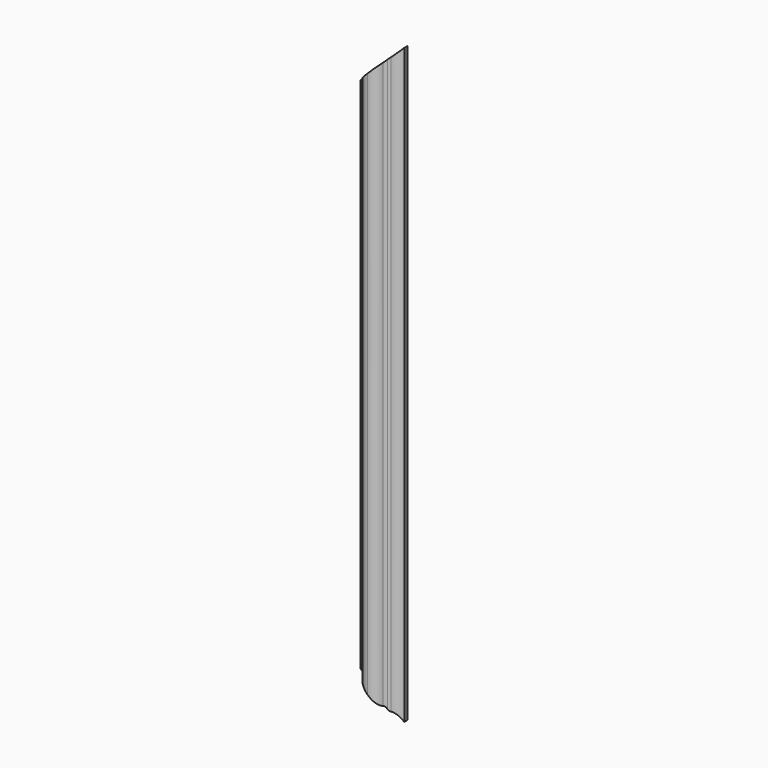
from build123d import *

# Parameters (mm, degrees)
F1_DEPTH = 250.825
F2_R     = 2.54
F3_R     = 2.54
F4_R     = 2.54
F6_W     = 6.35
F6_H     = 501.65
F7_DEPTH = 7.62
F8_DEPTH = 17.4635001


# Not quite as in the source:
# - ends of sketch curves that miss each other by under 0.0002 mm in the source are joined


with BuildPart() as f1:
    # F0 (on Top) → F1 (new body, symmetric)
    with BuildSketch(Plane.XY):
        with BuildLine():
            Line((15.875, 5.55625), (15.875, 8.73125))
            Line((15.875, 8.73125), (-15.875, 8.73125))
            Line((-15.875, 8.73125), (-15.875, -0.79375))
            Line((-15.875, -0.79375), (-12.7, -0.79375))
            ThreePointArc((-12.7, -0.79375), (-9.8710707302, -6.4481459867), (-3.9751, -8.73125))
            Line((-3.9751, -8.73125), (-3.96875, -8.73125))
            ThreePointArc((-3.96875, -8.73125), (1.9312218072, -6.4502821485), (4.7625, -0.79375))
            Line((4.7625, -0.79375), (7.9375, -0.79375))
            ThreePointArc((7.9375, -0.79375), (10.9883747468, 3.5285940665), (15.875, 5.55625))
        make_face()
    extrude(amount=F1_DEPTH, both=True)

    # F2
    f2_edges = [f1.edges().sort_by_distance(p)[0] for p in [
        (7.9375, -0.79375, 0),
    ]]
    fillet(f2_edges, radius=F2_R)

    # F3
    f3_edges = [f1.edges().sort_by_distance(p)[0] for p in [
        (-12.7, -0.79375, 0),
    ]]
    fillet(f3_edges, radius=F3_R)

    # F4
    f4_edges = [f1.edges().sort_by_distance(p)[0] for p in [
        (4.7625, -0.79375, 0),
    ]]
    fillet(f4_edges, radius=F4_R)

    # F6 (on face) → F7 (cut)
    with BuildSketch(Plane(origin=(0, 8.73125, 0), x_dir=(-1, 0, 0), z_dir=(0, 1, 0))):
        with Locations((12.7, 0)):
            Rectangle(F6_W, F6_H)
    extrude(amount=-F7_DEPTH, mode=Mode.SUBTRACT)

    # F5 (on face) → F8 (cut, through all)
    with BuildSketch(Plane(origin=(0, 8.73125, 0), x_dir=(-1, 0, 0), z_dir=(0, 1, 0))):
        Polygon((15.875, -250.825), (15.875, -219.075), (-15.875, -250.825), align=None)
        Polygon((-15.875, 250.825), (15.875, 219.075), (15.875, 250.825), align=None)
    extrude(amount=-F8_DEPTH, mode=Mode.SUBTRACT)


solid = f1.part
